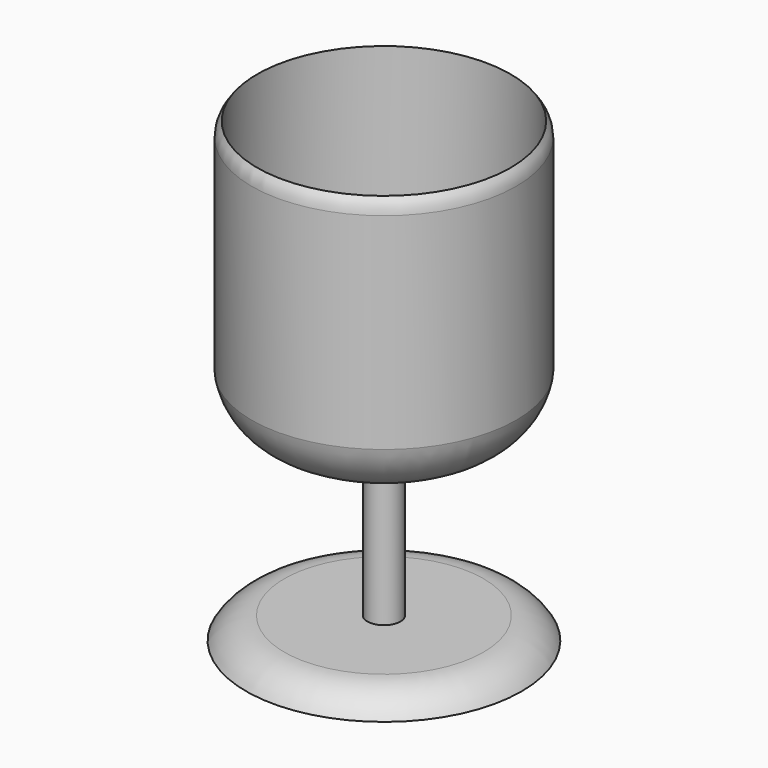
from build123d import *

# Parameters (mm, degrees)
F0_R     = 31.75
F1_DEPTH = 5.08
F3_R     = 3.81
F4_DEPTH = 49.53
F5_R     = 30.48
F5_R_2   = 3.81
F6_DEPTH = 50.8
F7_DEPTH = 12.7
F9_T     = -1.27


# Not quite as in the source:
# - a fillet or chamfer that OpenCascade refuses, or shapes differently, is made with other operations: its cross-section is extruded or revolved along the edge and cut away or added


with BuildPart() as f1:
    # F0 (on Top) → F1 (new body)
    with BuildSketch(Plane.XY):
        Circle(F0_R)
    extrude(amount=F1_DEPTH)

    # F2: fillet of radius 10.16 on 1 edges, made by hand

    # F2_s1 → F2_t2 (revolve, cut)
    with BuildSketch(Plane.XZ):
        with BuildLine():
            ThreePointArc((31.75, 0), (28.0311818975, 3.7188181024), (22.9511818975, 5.08))
            Line((22.9511818975, 5.08), (31.75, 5.08))
            Line((31.75, 5.08), (31.75, 0))
        make_face()
    revolve(axis=Axis((0, 0, 5.08), (0, 0, 1)), mode=Mode.SUBTRACT)

    # F3 (on face) → F4 (join)
    with BuildSketch(Plane.XY.offset(5.08)):
        Circle(F3_R)
    extrude(amount=F4_DEPTH)


with BuildPart() as f6:
    # F5 (on face) → F6 (new body)
    with BuildSketch(Plane.XY.offset(54.61)):
        Circle(F5_R)
        Circle(F5_R_2, mode=Mode.SUBTRACT)
    extrude(amount=F6_DEPTH)


with BuildPart() as f7:
    # F7 (new): a face of the model
    f7_faces = [f6.part.faces().sort_by_distance(p)[0] for p in [
        (-29.6178954124, 0, 54.61),
    ]]
    extrude(f7_faces, amount=F7_DEPTH)

    # F8: fillet of radius 15.24 on 1 edges, made by hand

    # F8_s1 → F8_t2 (revolve, cut)
    with BuildSketch(Plane.XZ):
        with BuildLine():
            ThreePointArc((30.48, 54.61), (25.2905350503, 45.5102577348), (15.4531573509, 41.91))
            Line((15.4531573509, 41.91), (30.48, 41.91))
            Line((30.48, 41.91), (30.48, 54.61))
        make_face()
    revolve(axis=Axis((0, 0, 41.91), (0, 0, 1)), mode=Mode.SUBTRACT)


with BuildPart() as f6_1:
    add(f6.part)

    # F9
    f9_openings = [f6_1.faces().sort_by_distance(p)[0] for p in [
        (-29.617895, 0, 105.41),
        (-3.81, 0, 80.01),
    ]]
    offset(amount=F9_T, openings=f9_openings)

    # F10: fillet of radius 5.08 on 1 edges, made by hand

    # F10_s1 → F10_t2 (revolve, cut)
    with BuildSketch(Plane.XZ):
        with BuildLine():
            ThreePointArc((30.48, 102.0498958349), (30.1519048812, 103.8459470592), (29.21, 105.41))
            Line((29.21, 105.41), (30.48, 105.41))
            Line((30.48, 105.41), (30.48, 102.0498958349))
        make_face()
    revolve(axis=Axis((0, 0, 105.41), (0, 0, 1)), mode=Mode.SUBTRACT)


solid = Compound([f1.part, f7.part, f6_1.part])
